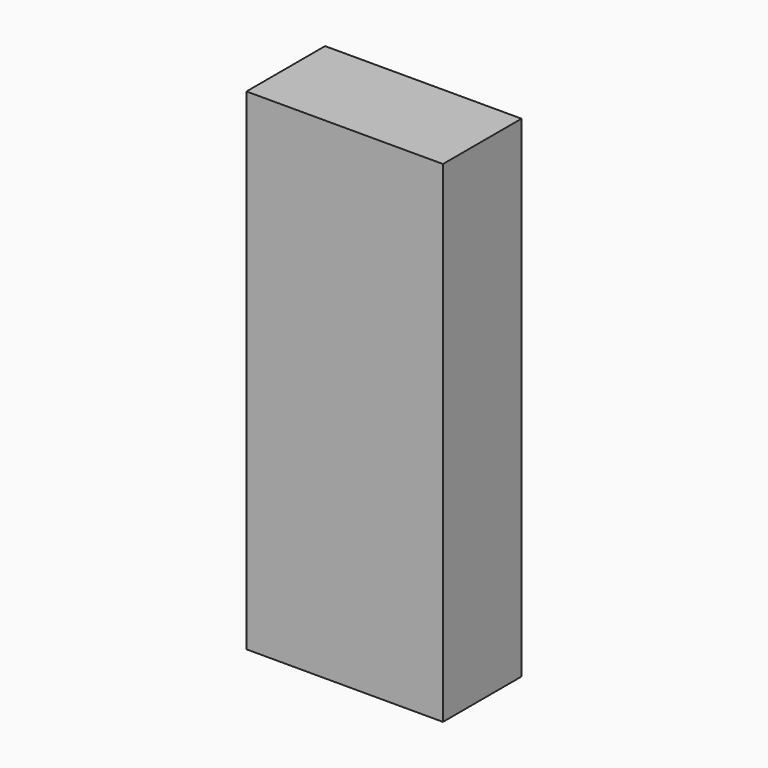
from build123d import *

# Parameters (mm, degrees)
F0_W     = 6.35
F0_H     = 15.875
F1_DEPTH = 3.175


# Not quite as in the source:
# - a length typed as a fraction of an inch, garbled in the dataset ("3 / 203.2 mm" for 3/8 in), is restored


with BuildPart() as f1:
    # F0 (on Front) → F1 (new body)
    with BuildSketch(Plane.XZ):
        Rectangle(F0_W, F0_H)
    extrude(amount=F1_DEPTH)


solid = f1.part
